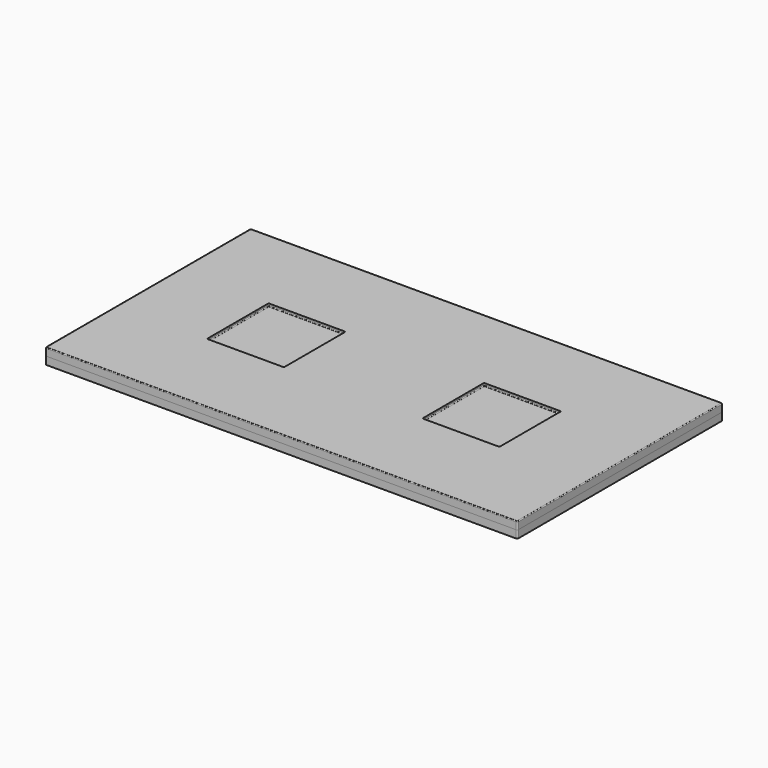
from build123d import *

# Parameters (mm, degrees)
F0_W         = 1840
F0_H         = 1000
F1_DEPTH     = 30
F2_W         = 300
F2_H         = 300
F3_DEPTH     = 10
F4_R         = 3
F5_T1_DEPTH  = 42.5
F5_T4_ANGLE  = 90
F5_T6_ANGLE  = 90
F5_T8_ANGLE  = 90
F5_T10_ANGLE = 90
F7_D         = 6
F7_DEPTH     = 18
F7_TIP       = 1.8025818571
F8_W         = 1720
F8_H         = 880
F9_DEPTH     = 30


# Not quite as in the source:
# - a fillet or chamfer that OpenCascade refuses, or shapes differently, is made with other operations: its cross-section is extruded or revolved along the edge and cut away or added


with BuildPart() as f1:
    # F0 (on Top) → F1 (new body)
    with BuildSketch(Plane.XY):
        with Locations((920, 500)):
            Rectangle(F0_W, F0_H)
    extrude(amount=F1_DEPTH)

    # F2 (on face) → F3 (cut)
    with BuildSketch(Plane.XY.offset(30)):
        with Locations((1340, 500)):
            Rectangle(F2_W, F2_H)
        with Locations((500, 500)):
            Rectangle(F2_W, F2_H)
    extrude(amount=-F3_DEPTH, mode=Mode.SUBTRACT)

    # F4
    f4_edges = [f1.edges().sort_by_distance(p)[0] for p in [
        (1490, 650, 25),
        (1190, 650, 25),
        (1190, 350, 25),
        (1490, 350, 25),
        (650, 650, 25),
        (350, 650, 25),
        (350, 350, 25),
        (650, 350, 25),
        (1340, 650, 20),
        (1190, 500, 20),
        (1340, 350, 20),
        (1490, 500, 20),
        (650, 500, 20),
        (500, 650, 20),
        (350, 500, 20),
        (500, 350, 20),
        (0, 500, 30),
        (920, 0, 30),
        (1840, 500, 30),
        (920, 1000, 30),
    ]]
    fillet(f4_edges, radius=F4_R)

    # F5: fillet of radius 5 on 4 edges, made by hand

    # F5_s2 → F5_t1 (cut)
    with BuildSketch(Plane.XY.offset(-12.5)):
        with BuildLine():
            ThreePointArc((1835, 1000), (1838.5355339059, 998.5355339059), (1840, 995))
            Line((1840, 995), (1840, 1000))
            Line((1840, 1000), (1835, 1000))
        make_face()
        with BuildLine():
            ThreePointArc((1835, 0), (1838.5355339059, 1.4644660941), (1840, 5))
            Line((1840, 5), (1840, 0))
            Line((1840, 0), (1835, 0))
        make_face()
        with BuildLine():
            ThreePointArc((0, 5), (1.4644660941, 1.4644660941), (5, 0))
            Line((5, 0), (0, 0))
            Line((0, 0), (0, 5))
        make_face()
        with BuildLine():
            ThreePointArc((0, 995), (1.4644660941, 998.5355339059), (5, 1000))
            Line((5, 1000), (0, 1000))
            Line((0, 1000), (0, 995))
        make_face()
    extrude(amount=F5_T1_DEPTH, mode=Mode.SUBTRACT)

    # F5_s3 → F5_t4 (revolve, cut)
    with BuildSketch(Plane.YZ.offset(5)):
        with BuildLine():
            ThreePointArc((997, 30), (999.1213203436, 29.1213203436), (1000, 27))
            Line((1000, 27), (1000, 30))
            Line((1000, 30), (997, 30))
        make_face()
    revolve(axis=Axis((5, 995, 30), (0, 0, 1)), revolution_arc=F5_T4_ANGLE, mode=Mode.SUBTRACT)

    # F5_s5 → F5_t6 (revolve, cut)
    with BuildSketch(Plane.XZ.offset(-5)):
        with BuildLine():
            ThreePointArc((3, 30), (0.8786796564, 29.1213203436), (0, 27))
            Line((0, 27), (0, 30))
            Line((0, 30), (3, 30))
        make_face()
    revolve(axis=Axis((5, 5, 30), (0, 0, 1)), revolution_arc=F5_T6_ANGLE, mode=Mode.SUBTRACT)

    # F5_s7 → F5_t8 (revolve, cut)
    with BuildSketch(Plane.YZ.offset(1835)):
        with BuildLine():
            ThreePointArc((3, 30), (0.8786796564, 29.1213203436), (0, 27))
            Line((0, 27), (0, 30))
            Line((0, 30), (3, 30))
        make_face()
    revolve(axis=Axis((1835, 5, 30), (0, 0, 1)), revolution_arc=F5_T8_ANGLE, mode=Mode.SUBTRACT)

    # F5_s9 → F5_t10 (revolve, cut)
    with BuildSketch(Plane.XZ.offset(-995)):
        with BuildLine():
            ThreePointArc((1837, 30), (1839.1213203436, 29.1213203436), (1840, 27))
            Line((1840, 27), (1840, 30))
            Line((1840, 30), (1837, 30))
        make_face()
    revolve(axis=Axis((1835, 995, 30), (0, 0, 1)), revolution_arc=F5_T10_ANGLE, mode=Mode.SUBTRACT)

    # F7
    with Locations(Plane(origin=(0, 0, 0), x_dir=(1, 0, 0), z_dir=(0, 0, -1))):
        with Locations((325, -325), (675, -325), (325, -675), (675, -675), (1165, -675), (1165, -325), (1515, -325), (1515, -675)):
            Hole(F7_D / 2, depth=F7_DEPTH)
            with Locations((0, 0, -(F7_DEPTH + F7_TIP / 2))):  # 118° drill point
                Cone(0, F7_D / 2, F7_TIP, mode=Mode.SUBTRACT)


with BuildPart() as f9:
    # F8 (on face) → F9 (new body)
    with BuildSketch(Plane(origin=(0, 0, 0), x_dir=(1, 0, 0), z_dir=(0, 0, -1))):
        with BuildLine():
            Line((1835, 0), (5, 0))
            ThreePointArc((5, 0), (1.4644660941, -1.4644660941), (0, -5))
            Line((0, -5), (0, -995))
            ThreePointArc((0, -995), (1.4644660941, -998.5355339059), (5, -1000))
            Line((5, -1000), (1835, -1000))
            ThreePointArc((1835, -1000), (1838.5355339059, -998.5355339059), (1840, -995))
            Line((1840, -995), (1840, -5))
            ThreePointArc((1840, -5), (1838.5355339059, -1.4644660941), (1835, 0))
        make_face()
        with Locations((920, -500)):
            Rectangle(F8_W, F8_H, mode=Mode.SUBTRACT)
    extrude(amount=F9_DEPTH)


solid = Compound([f1.part, f9.part])
